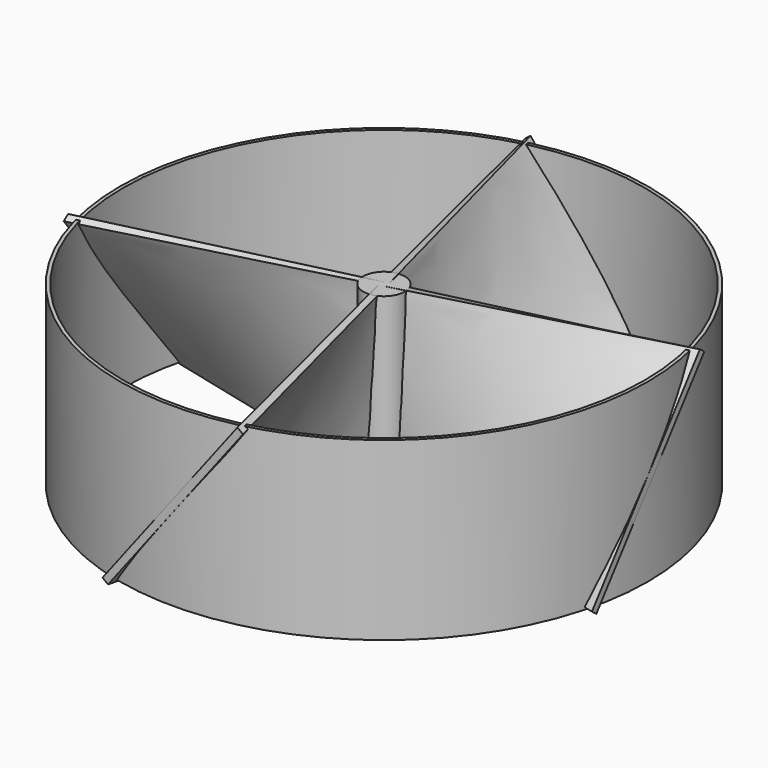
from build123d import *

# Parameters (mm, degrees)
F0_R      = 76.2
F0_R_2    = 75.2
F1_DEPTH  = 50.8
F7_W      = 2
F7_H      = 50.8
F9_COUNT  = 4
F10_R     = 6
F11_DEPTH = 50.8


# Not quite as in the source:
# - a feature of the source that left no trace in its solid (it failed there, or was rolled back) is left out
# - the program builds the solid bodies; features that only make, move or delete a surface that nothing else refers to are left out


with BuildPart() as f1:
    # F0 (on Top) → F1 (new body)
    with BuildSketch(Plane.XY):
        Circle(F0_R)
        Circle(F0_R_2, mode=Mode.SUBTRACT)
    extrude(amount=F1_DEPTH)


with BuildPart() as f8:
    # F7 (on Right) → F8 section 0
    with BuildSketch(Plane.YZ):
        with Locations((0, 25.4)):
            Rectangle(F7_W, F7_H)
    # F6 (on offset) → F8 section 1
    with BuildSketch(Plane.YZ.offset(-76.2)):
        Polygon((20.2569515517, 0.6082319282), (-18.6694328318, 51.4082319282), (-20.2569515517, 50.1917680718), (18.6694328318, -0.6082319282), align=None)
    loft()


with BuildPart() as f9_1:
    # F9: instance of F8
    add(f8.part.rotate(Axis((0, 0, 31.0026016086), (0, 0, 1)), 1 * 360 / F9_COUNT))


with BuildPart() as f9_2:
    # F9: instance of F8
    add(f8.part.rotate(Axis((0, 0, 31.0026016086), (0, 0, 1)), 2 * 360 / F9_COUNT))


with BuildPart() as f9_3:
    # F9: instance of F8
    add(f8.part.rotate(Axis((0, 0, 31.0026016086), (0, 0, 1)), 3 * 360 / F9_COUNT))


with BuildPart() as f11:
    # F10 (on Top) → F11 (new body, through all)
    with BuildSketch(Plane.XY):
        Circle(F10_R)
    extrude(amount=F11_DEPTH)


solid = Compound([f1.part, f8.part, f9_1.part, f9_2.part, f9_3.part, f11.part])
